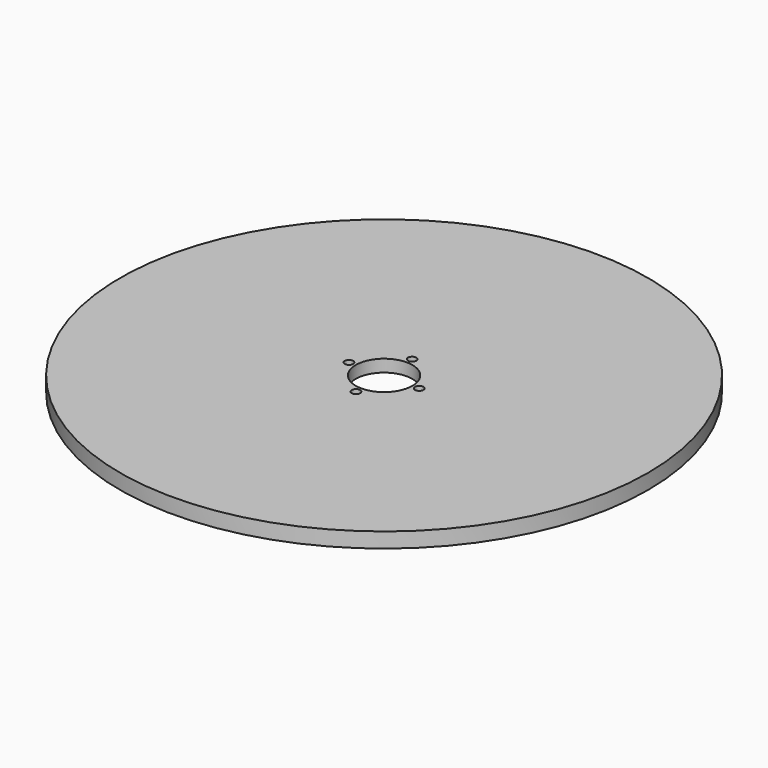
from build123d import *

# Parameters (mm, degrees)
F0_R     = 280
F1_DEPTH = 16
F2_R     = 30
F2_R_2   = 4.5
F3_DEPTH = 25
F4_R     = 44.25
F4_R_2   = 4.5
F4_R_3   = 30
F5_DEPTH = 3


# Not quite as in the source:
# - a feature names something its author has since deleted; it is built from what else it names


with BuildPart() as f1:
    # F0 (on Top) → F1 (new body)
    with BuildSketch(Plane.XY):
        Circle(F0_R)
    extrude(amount=F1_DEPTH)

    # F2 (on face) → F3 (cut)
    with BuildSketch(Plane.XY.offset(16)):
        Circle(F2_R)
        with Locations((-37.25, 0)):
            Circle(F2_R_2)
        with Locations((0, 37.25)):
            Circle(F2_R_2)
        with Locations((37.25, 0)):
            Circle(F2_R_2)
        with Locations((0, -37.25)):
            Circle(F2_R_2)
    extrude(amount=-F3_DEPTH, mode=Mode.SUBTRACT)

    # F4 (on face) → F5 (cut)
    with BuildSketch(Plane(origin=(0, 0, 0), x_dir=(1, 0, 0), z_dir=(0, 0, -1))):
        Circle(F4_R)
        with Locations((0, -37.25)):
            Circle(F4_R_2, mode=Mode.SUBTRACT)
        with Locations((-37.25, 0)):
            Circle(F4_R_2, mode=Mode.SUBTRACT)
        Circle(F4_R_3, mode=Mode.SUBTRACT)
        with Locations((37.25, 0)):
            Circle(F4_R_2, mode=Mode.SUBTRACT)
        with Locations((0, 37.25)):
            Circle(F4_R_2, mode=Mode.SUBTRACT)
    extrude(amount=-F5_DEPTH, mode=Mode.SUBTRACT)


solid = f1.part
